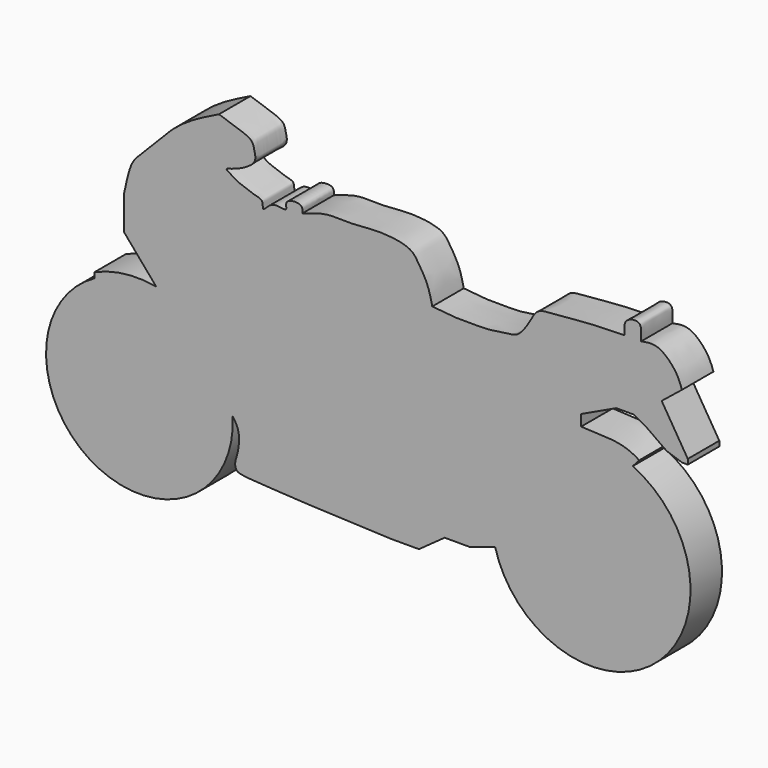
from build123d import *

# Parameters (mm, degrees)
F2_DEPTH  = 10
F14_SCALE = 0.5


# Not quite as in the source:
# - a feature names something its author has since deleted; it is built from what else it names
# - the program builds the solid bodies; features that only make, move or delete a surface that nothing else refers to are left out


with BuildPart() as f2:
    # F0 (on Front) → F2 (new body)
    with BuildSketch(Plane.XZ):
        with BuildLine():
            Line((-70.1603144407, 2.7968266513), (-70.1603144407, 1.4234187547))
            ThreePointArc((-70.1603144407, 1.4234187547), (-70.2145489266, -40.1372623928), (-35.0422821939, -17.99669303))
            add(Edge.make_bspline(
                [(-15.8571563661, -31.4765945077), (-18.7177282322, -31.3101976564), (-24.2975162547, -30.9856264864), (-32.7728139412, -30.5720339527), (-34.1921223492, -29.8256076047), (-34.6083105275, -28.1678758484), (-33.5909596521, -25.8280983966), (-33.1225179299, -20.7680472143), (-34.4474763908, -18.8553492631), (-35.0422821939, -17.99669303)],
                knots=[0, 0, 0, 0, 0.2173047805, 0.4238714034, 0.5069732944, 0.59224959, 0.7085549741, 0.8691633, 1, 1, 1, 1], degree=3))
            Line((-15.8571563661, -31.4765945077), (5.1956321113, -32.3513820767))
            Line((5.1956321113, -32.3513820767), (12.2905466706, -32.3513820767))
            Line((12.2905466706, -32.3513820767), (18.8132897019, -27.6581868529))
            Line((18.8132897019, -27.6581868529), (25.2216011286, -27.6581868529))
            Line((25.2216011286, -27.6581868529), (31.6383130848, -25.5408957601))
            ThreePointArc((31.6383130848, -25.5408957601), (72.3006146402, -38.3663180252), (66.61169976, 3.8894563913))
            Line((66.61169976, 3.8894563913), (68.254083395, 5.7316944003))
            add(Edge.make_bspline(
                [(53.5132065415, 8.4772780538), (55.5040504231, 8.3929973978), (59.1229435492, 8.2397946834), (62.8884494062, 8.0039185472), (66.2136316185, 7.0026107145), (67.6151226177, 6.1296776731), (68.254083395, 5.7316944003)],
                knots=[0, 0, 0, 0, 0.309506582, 0.5626112888, 0.8005879231, 1, 1, 1, 1], degree=3))
            Line((53.5132065415, 8.4772780538), (53.5132065415, 11.2915560603))
            Line((53.5132065415, 11.2915560603), (62.4142251909, 15.5102163553))
            Line((62.4142251909, 15.5102163553), (66.8887943029, 15.5102163553))
            Line((66.8887943029, 15.5102163553), (69.8718354106, 13.8771906495))
            Line((69.8718354106, 13.8771906495), (75.2605646849, 10.0667849183))
            Line((75.2605646849, 10.0667849183), (79.1111662984, 8.7739676237))
            Line((79.1111662984, 8.7739676237), (80.6011706591, 8.7739676237))
            Line((80.6011706591, 8.7739676237), (80.6011706591, 10.0667849183))
            Line((80.6011706591, 10.0667849183), (73.9614963531, 20.8856090903))
            Line((73.9614963531, 20.8856090903), (79.1111662984, 25.0245854259))
            add(Edge.make_bspline(
                [(68.7471404672, 32.5022675097), (70.1725898279, 32.7793130486), (73.2938248363, 33.3859457769), (77.916531806, 28.5701341988), (78.7465965554, 26.1065898492), (79.1111662984, 25.0245854259)],
                knots=[0, 0, 0, 0, 0.320372303, 0.7015031719, 1, 1, 1, 1], degree=3))
            add(Edge.make_bspline(
                [(64.5394474268, 32.5022675097), (64.4678746972, 33.3281659297), (64.3336751663, 34.8767331162), (65.3074974299, 36.583257466), (68.9348334976, 37.0546546226), (68.7159394615, 33.752163088), (68.7379893371, 32.8688568812), (68.7471404672, 32.5022675097)],
                knots=[0, 0, 0, 0, 0.2110428468, 0.3957072923, 0.6208524643, 0.8426463487, 1, 1, 1, 1], degree=3))
            add(Edge.make_bspline(
                [(15.6742297113, 23.0450052768), (16.5844261538, 22.950517427), (18.5416596475, 22.7473362503), (22.2134815433, 22.3813790317), (26.7425739772, 22.5076492148), (30.0673752989, 22.4221219429), (33.0687156287, 23.1330233641), (36.7484371708, 23.3396420412), (37.7837193781, 24.1910856931), (38.7803693746, 25.1853678195), (40.0816926768, 27.0530140531), (41.1038373203, 28.9739302108), (41.8159494962, 30.0810432773), (43.1494936511, 31.2259085067), (46.3483660216, 31.3512583703), (49.825758526, 31.617249819), (54.7691971013, 32.2507714382), (60.915638935, 32.4089870339), (64.5394474268, 32.5022675097)],
                knots=[0, 0, 0, 0, 0.0602109997, 0.1294742319, 0.206125857, 0.2710327483, 0.3350993906, 0.4027209808, 0.442562564, 0.4841366051, 0.5387808948, 0.5918687573, 0.632417919, 0.6776597614, 0.7406666278, 0.8075501518, 0.886535753, 1, 1, 1, 1], degree=3))
            add(Edge.make_bspline(
                [(-17.3478778452, 33.1136696041), (-16.7450423087, 33.3235113693), (-15.2765292766, 33.8346878815), (-10.8404654954, 35.2485304708), (-6.6181952167, 34.6630061736), (1.0225500837, 35.4682293276), (5.8986738705, 35.2319050649), (10.5021919637, 34.1876461101), (12.1038937154, 31.6764601114), (13.9997454046, 28.7017140278), (15.0060882242, 26.0327120836), (15.4493929289, 24.0504006879), (15.6742297113, 23.0450052768)],
                knots=[0, 0, 0, 0, 0.0741099478, 0.1805325293, 0.28726009, 0.4261434308, 0.5413357632, 0.6463970839, 0.7316677568, 0.8260877502, 0.9117945958, 1, 1, 1, 1], degree=3))
            add(Edge.make_bspline(
                [(-38.5178700089, 48.413798213), (-37.2086618929, 47.9310095594), (-34.5880423183, 46.9646197389), (-29.9615394566, 45.6999431744), (-29.6125265988, 43.4299128331), (-29.1240780119, 41.6873723706), (-29.6061919281, 40.2143165806), (-31.3477649295, 39.0287920321), (-32.6152258482, 38.2767963146), (-35.0993510451, 37.2129778975), (-37.2117205405, 36.8799871988), (-35.2378339505, 35.8285430158), (-33.8539497276, 34.8614651493), (-31.5699444534, 34.0837040019), (-29.1125300687, 33.1600673113), (-27.1965479006, 32.8675475679), (-27.6060878868, 30.0347312892), (-25.7306387383, 32.44701128), (-23.8437548611, 32.9672791313), (-20.8263691722, 32.1281067533), (-22.2164084081, 35.0023418104), (-17.1508415545, 35.4666855058), (-17.2898376362, 33.8067882885), (-17.3478778452, 33.1136696041)],
                knots=[0, 0, 0, 0, 0.0680352424, 0.1361849854, 0.1819600343, 0.2250268681, 0.2638982165, 0.3096732947, 0.3501564903, 0.4054524889, 0.4430780006, 0.4821240757, 0.5268973467, 0.5770004087, 0.6307843783, 0.6723521021, 0.7130285408, 0.7572149163, 0.8066475228, 0.8539346518, 0.8956454287, 0.9564249506, 1, 1, 1, 1], degree=3))
            add(Edge.make_bspline(
                [(-62.5952631235, 23.0450052768), (-62.3848416036, 24.0428871056), (-61.9419178755, 26.1433639955), (-60.9223040871, 30.0290599328), (-59.4685270888, 31.9650102976), (-57.2850306102, 34.1952396219), (-54.7934110836, 36.5511024905), (-48.8073579355, 43.3714030755), (-42.1151835801, 46.6509236571), (-38.5178700089, 48.413798213)],
                knots=[0, 0, 0, 0, 0.1174395667, 0.2472027136, 0.3492573428, 0.4612870362, 0.5820754532, 0.7753487037, 1, 1, 1, 1], degree=3))
            Line((-62.5952631235, 23.0450052768), (-62.5952631235, 14.1441216692))
            Line((-62.5952631235, 14.1441216692), (-54.4623918831, 4.6601039357))
            ThreePointArc((-54.4623918831, 4.6601039357), (-62.4531100103, 4.922752395), (-70.1603144407, 2.7968266513))
        make_face()
    extrude(amount=-F2_DEPTH)


with BuildPart() as f2_1:
    # F14: moved
    add(f2.part.scale(F14_SCALE).moved(Location((-19.2589350045, 0, 24.2068991065))))


solid = f2_1.part
